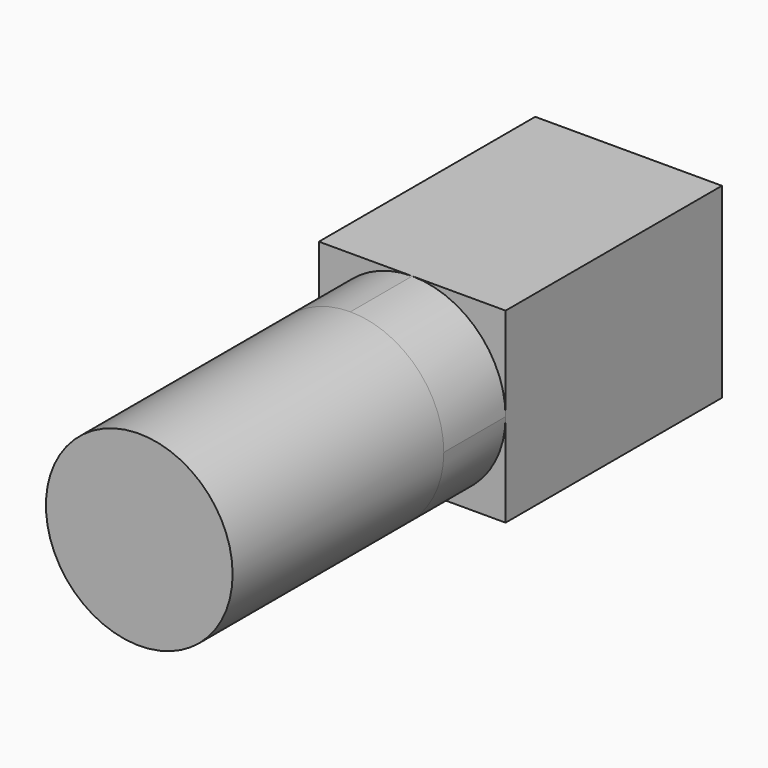
from build123d import *

# Parameters (mm, degrees)
F0_W     = 29
F0_H     = 42
F1_DEPTH = 29
F3_DEPTH = 12
F4_R     = 14.5
F5_DEPTH = 41


# Not quite as in the source:
# - the program builds the solid bodies; features that only make, move or delete a surface that nothing else refers to are left out


with BuildPart() as f1:
    # F0 (on Top) → F1 (new body)
    with BuildSketch(Plane.XY):
        Rectangle(F0_W, F0_H)
    extrude(amount=F1_DEPTH)

    # F2 (on face) → F3 (join)
    with BuildSketch(Plane.XZ.offset(21)):
        with BuildLine():
            ThreePointArc((0, 0), (10.2530483272, 4.2469516728), (14.5, 14.5))
            ThreePointArc((14.5, 14.5), (10.2530483272, 24.7530483272), (0, 29))
            ThreePointArc((0, 29), (-10.2530483272, 24.7530483272), (-14.5, 14.5))
            ThreePointArc((-14.5, 14.5), (-10.2530483272, 4.2469516728), (0, 0))
        make_face()
    extrude(amount=F3_DEPTH)

    # F4 (on face) → F5 (join)
    with BuildSketch(Plane.XZ.offset(33)):
        with Locations((0, 14.5)):
            Circle(F4_R)
    extrude(amount=F5_DEPTH)


solid = f1.part
